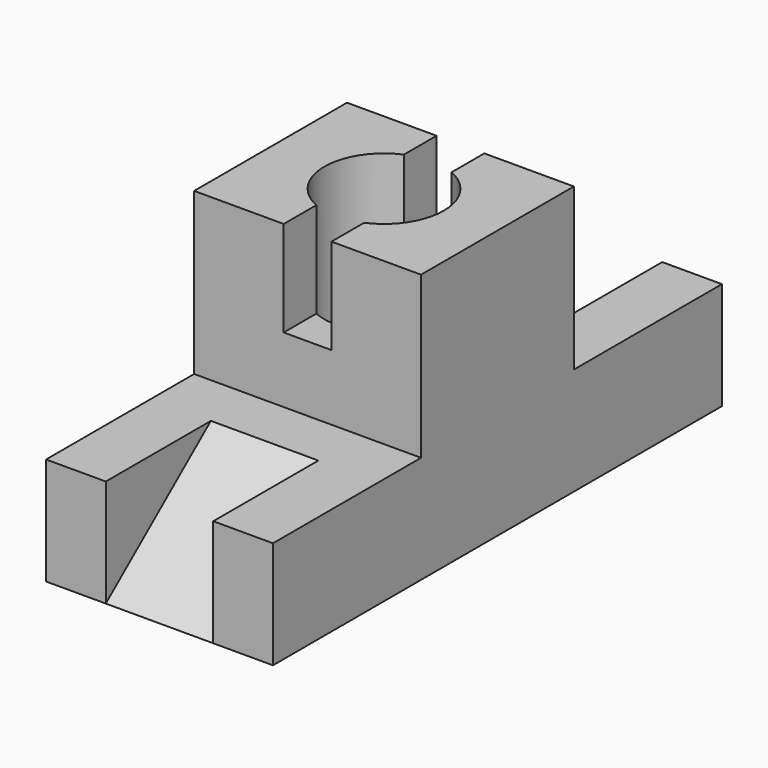
from build123d import *

# Parameters (mm, degrees)
F0_W     = 94
F0_H     = 45
F1_DEPTH = 19
F2_W     = 31
F2_H     = 27
F3_DEPTH = 38.001
F4_R     = 10
F5_DEPTH = 45.001
F6_W     = 8
F6_H     = 32
F7_DEPTH = 16
F9_DEPTH = 9


# Not quite as in the source:
# - a pattern or mirror of a feature is missing from the dataset's text; its kind, count and spacing are read off the source's solid


with BuildPart() as f1:
    # F0 (on Right) → F1 (new body, symmetric)
    with BuildSketch(Plane.YZ):
        Rectangle(F0_W, F0_H)
    extrude(amount=F1_DEPTH, both=True)

    # F2 (on face) → F3 (cut, through all)
    with BuildSketch(Plane.YZ.offset(19)):
        with Locations((-31.5, 9)):
            Rectangle(F2_W, F2_H)
    f3 = extrude(amount=-F3_DEPTH, mode=Mode.SUBTRACT)

    # F3_copies: F3 across plane
    add(f3.mirror(Plane.ZX), mode=Mode.SUBTRACT)

    # F4 (on face) → F5 (cut, through all)
    with BuildSketch(Plane.XY.offset(22.5)):
        Circle(F4_R)
    extrude(amount=-F5_DEPTH, mode=Mode.SUBTRACT)

    # F6 (on face) → F7 (cut)
    with BuildSketch(Plane.XY.offset(22.5)):
        Rectangle(F6_W, F6_H)
    extrude(amount=-F7_DEPTH, mode=Mode.SUBTRACT)

    # F8 (on Right) → F9 (cut, symmetric)
    with BuildSketch(Plane.YZ):
        Polygon((-25, -4.5), (-47, -4.5), (-47, -22.5), align=None)
    f9 = extrude(amount=F9_DEPTH, both=True, mode=Mode.SUBTRACT)

    # F9_copies: F9 across plane
    add(f9.mirror(Plane.ZX), mode=Mode.SUBTRACT)


solid = f1.part
